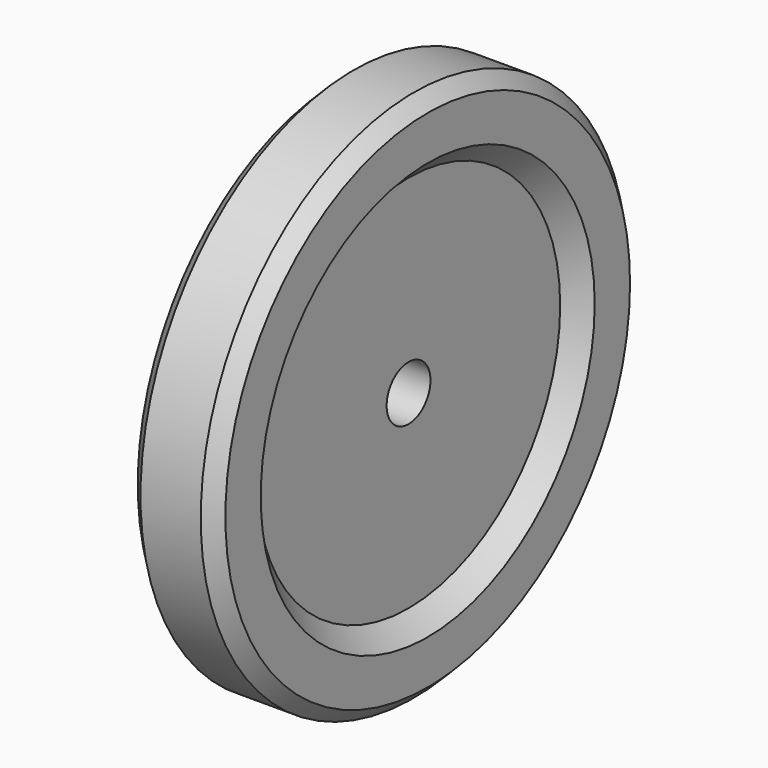
from build123d import *

# Parameters (mm, degrees)
F0_R     = 66.2228003741
F0_R_2   = 10
F1_DEPTH = 25
F0_R_3   = 97.356020809
F0_R_4   = 74.349079459
F2_DEPTH = 32
F4_SIZE  = 5
F5_SIZE  = 5


# Not quite as in the source:
# - a fillet or chamfer that OpenCascade refuses, or shapes differently, is made with other operations: its cross-section is extruded or revolved along the edge and cut away or added


with BuildPart() as f1:
    # F0 (on Right) → F1 (new body)
    with BuildSketch(Plane.YZ):
        Circle(F0_R)
        Circle(F0_R_2, mode=Mode.SUBTRACT)
    extrude(amount=F1_DEPTH)

    # F0 (on Right) → F2 (join)
    with BuildSketch(Plane.YZ):
        Circle(F0_R_3)
        Circle(F0_R_4, mode=Mode.SUBTRACT)
        Circle(F0_R_4)
        Circle(F0_R, mode=Mode.SUBTRACT)
    extrude(amount=F2_DEPTH)

    # F3: chamfer of 10 on 1 edges, made by hand


with BuildPart() as f3_tool2:
    # F3_s3 → F3_t4 (revolve)
    with BuildSketch(Plane.XY):
        Polygon((22, 66.2228003741), (32, 76.2228003741), (32, 66.2228003741), align=None)
    revolve(axis=Axis((32, 0, 0), (1, 0, 0)))

    split(bisect_by=Plane.YZ.offset(25), keep=Keep.TOP)


with BuildPart() as f1_1:
    add(f1.part)

    # F3_t1: cut F3_tool2
    add(f3_tool2.part, mode=Mode.SUBTRACT)

    # F4
    f4_edges = [f1_1.edges().sort_by_distance(p)[0] for p in [
        (32, -97.356021, 0),
    ]]
    chamfer(f4_edges, length=F4_SIZE)

    # F5
    f5_edges = [f1_1.edges().sort_by_distance(p)[0] for p in [
        (0, -97.356021, 0),
    ]]
    chamfer(f5_edges, length=F5_SIZE)


solid = f1_1.part
